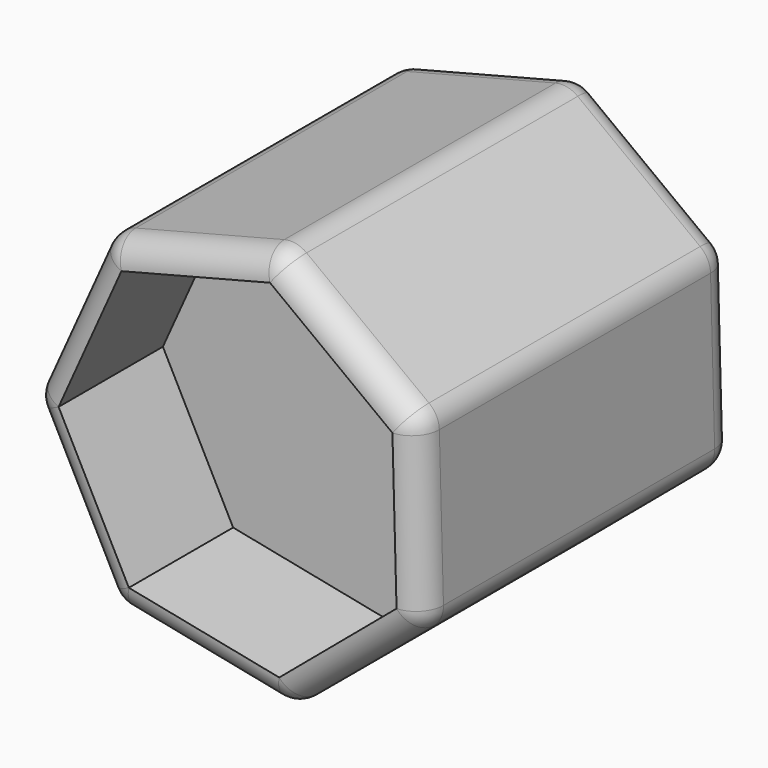
from build123d import *

# Parameters (mm, degrees)
F1_DEPTH     = 76.2
F2_F1_R      = 5.08
F2_F2_R      = 5.08
F2_F3_R      = 5.08
F2_F4_R      = 5.08
F3_T1_DEPTH  = 66.04
F3_T3_DEPTH  = 29.883199232
F3_T5_DEPTH  = 29.883199232
F3_T7_DEPTH  = 29.883199232
F3_T9_DEPTH  = 29.883199232
F3_T14_DEPTH = 5.08
F3_T20_DEPTH = 5.08
F3_T26_DEPTH = 5.08
F3_T32_DEPTH = 5.08
F3_T38_DEPTH = 5.08
F3_T44_DEPTH = 5.08
F3_T50_DEPTH = 5.08
F3_T56_DEPTH = 5.08
F3_T62_DEPTH = 5.08
F3_T68_DEPTH = 5.08
F5_DEPTH     = 25.4
F6_DEPTH     = 25.4


# Not quite as in the source:
# - a fillet or chamfer that OpenCascade refuses, or shapes differently, is made with other operations: its cross-section is extruded or revolved along the edge and cut away or added
# - a feature of the source that left no trace in its solid (it failed there, or was rolled back) is left out


with BuildPart() as f1:
    # F0 (on Front) → F1 (new body)
    with BuildSketch(Plane.XZ):
        Polygon((36.5605491077, -17.381725656), (35.6265013603, 17.381725656), (7.8649714404, 38.3261150914), (-25.8190423903, 29.6798902177), (-40.0607906887, -2.0461652844), (-24.1359465072, -32.9616845282), (9.9637576777, -39.7866509615), align=None)
    extrude(amount=F1_DEPTH)

    # F2: fillet of radius 5.08 on 4 edges, made by hand

    # F2_f1
    f2_f1_edges = [f1.edges().sort_by_distance(p)[0] for p in [
        (7.8649714404, -38.1, 38.3261150914),
    ]]
    fillet(f2_f1_edges, radius=F2_F1_R)

    # F2_f2
    f2_f2_edges = [f1.edges().sort_by_distance(p)[0] for p in [
        (-25.8190423903, -38.1, 29.6798902177),
    ]]
    fillet(f2_f2_edges, radius=F2_F2_R)

    # F2_f3
    f2_f3_edges = [f1.edges().sort_by_distance(p)[0] for p in [
        (-8.9770354749, 0, 34.0030026545),
    ]]
    fillet(f2_f3_edges, radius=F2_F3_R)

    # F2_f4
    f2_f4_edges = [f1.edges().sort_by_distance(p)[0] for p in [
        (-8.9770354749, -76.2, 34.0030026545),
    ]]
    fillet(f2_f4_edges, radius=F2_F4_R)

    # F3: fillet of radius 5.08 on 19 edges, made by hand

    # F3_s2 → F3_t1 (cut)
    with BuildSketch(Plane.XZ.offset(5.08)):
        with BuildLine():
            ThreePointArc((35.6922091389, 14.9362091735), (35.1301118192, 17.1260312252), (33.6735514536, 18.8551078331))
            Line((33.6735514536, 18.8551078331), (35.6265013603, 17.381725656))
            Line((35.6265013603, 17.381725656), (35.6922091389, 14.9362091735))
        make_face()
        with BuildLine():
            ThreePointArc((34.6895354607, -18.957852653), (36.0511453352, -17.1530555552), (36.4948413291, -14.9362091735))
            Line((36.4948413291, -14.9362091735), (36.5605491077, -17.381725656))
            Line((36.5605491077, -17.381725656), (34.6895354607, -18.957852653))
        make_face()
        with BuildLine():
            ThreePointArc((7.564934043, -39.3065326972), (9.8249311044, -39.245809579), (11.8347713247, -38.2105239645))
            Line((11.8347713247, -38.2105239645), (9.9637576777, -39.7866509615))
            Line((9.9637576777, -39.7866509615), (7.564934043, -39.3065326972))
        make_face()
        with BuildLine():
            ThreePointArc((-25.2562170056, -30.7868598483), (-23.79965664, -32.5159364562), (-21.7371228725, -33.4418027925))
            Line((-21.7371228725, -33.4418027925), (-24.1359465072, -32.9616845282))
            Line((-24.1359465072, -32.9616845282), (-25.2562170056, -30.7868598483))
        make_face()
        with BuildLine():
            ThreePointArc((-38.9405201903, -4.2209899644), (-39.50261751, -2.0311679128), (-39.0589215161, 0.1856784689))
            Line((-39.0589215161, 0.1856784689), (-40.0607906887, -2.0461652844))
            Line((-40.0607906887, -2.0461652844), (-38.9405201903, -4.2209899644))
        make_face()
    extrude(amount=F3_T1_DEPTH, mode=Mode.SUBTRACT)

    # F3_s4 → F3_t3 (cut)
    with BuildSketch(Plane(origin=(0.4273541338, 0, -15.9052946325), x_dir=(0, 1, 0), z_dir=(-0.026858978, 0, 0.9996392326))):
        with BuildLine():
            ThreePointArc((-76.2, -31.0005038658), (-74.7121024484, -34.5926063143), (-71.12, -36.0805038658))
            Line((-71.12, -36.0805038658), (-76.2, -36.0805038658))
            Line((-76.2, -36.0805038658), (-76.2, -31.0005038658))
        make_face()
        with BuildLine():
            ThreePointArc((0, -31.0005038658), (-1.4878975516, -34.5926063143), (-5.08, -36.0805038658))
            Line((-5.08, -36.0805038658), (0, -36.0805038658))
            Line((0, -36.0805038658), (0, -31.0005038658))
        make_face()
    extrude(amount=F3_T3_DEPTH, mode=Mode.SUBTRACT)

    # F3_s6 → F3_t5 (cut)
    with BuildSketch(Plane(origin=(-11.9052292748, 0, -10.0288703376), x_dir=(0, 1, 0), z_dir=(0.7648031243, 0, 0.6442640616))):
        with BuildLine():
            ThreePointArc((0, -31.7682459503), (-1.4878975516, -35.3603483987), (-5.08, -36.8482459503))
            Line((-5.08, -36.8482459503), (0, -36.8482459503))
            Line((0, -36.8482459503), (0, -31.7682459503))
        make_face()
        with BuildLine():
            ThreePointArc((-76.2, -31.7682459503), (-74.7121024484, -35.3603483987), (-71.12, -36.8482459503))
            Line((-71.12, -36.8482459503), (-76.2, -36.8482459503))
            Line((-76.2, -36.8482459503), (-76.2, -31.7682459503))
        make_face()
    extrude(amount=F3_T5_DEPTH, mode=Mode.SUBTRACT)

    # F3_s8 → F3_t7 (cut)
    with BuildSketch(Plane(origin=(-14.4644044829, 0, 2.8950126528), x_dir=(0, 1, 0), z_dir=(0.9805528748, 0, -0.1962550883))):
        with BuildLine():
            ThreePointArc((0, -31.9774768364), (-1.4878975516, -35.5695792849), (-5.08, -37.0574768364))
            Line((-5.08, -37.0574768364), (0, -37.0574768364))
            Line((0, -37.0574768364), (0, -31.9774768364))
        make_face()
        with BuildLine():
            ThreePointArc((-76.2, -31.9774768364), (-74.7121024484, -35.5695792849), (-71.12, -37.0574768364))
            Line((-71.12, -37.0574768364), (-76.2, -37.0574768364))
            Line((-76.2, -37.0574768364), (-76.2, -31.9774768364))
        make_face()
    extrude(amount=F3_T7_DEPTH, mode=Mode.SUBTRACT)

    # F3_s10 → F3_t9 (cut)
    with BuildSketch(Plane(origin=(-6.4473598679, 0, 12.5165104158), x_dir=(0, 1, 0), z_dir=(0.457926311, 0, -0.8889901539))):
        with BuildLine():
            ThreePointArc((-71.12, -36.5506413995), (-74.7121024484, -35.0627438479), (-76.2, -31.4706413995))
            Line((-76.2, -31.4706413995), (-76.2, -36.5506413995))
            Line((-76.2, -36.5506413995), (-71.12, -36.5506413995))
        make_face()
        with BuildLine():
            ThreePointArc((-5.08, -36.5506413995), (-1.4878975516, -35.0627438479), (0, -31.4706413995))
            Line((0, -31.4706413995), (0, -36.5506413995))
            Line((0, -36.5506413995), (-5.08, -36.5506413995))
        make_face()
    extrude(amount=F3_T9_DEPTH, mode=Mode.SUBTRACT)


with BuildPart() as f3_tool12:
    # F3_s13 → F3_t14 (new body)
    with BuildSketch(Plane.XZ.offset(71.12)):
        Polygon((30.6140418374, 14.7997655654), (35.6922091389, 14.9362091735), (35.6265013603, 17.381725656), (33.6735514536, 18.8551078331), align=None)
    extrude(amount=F3_T14_DEPTH)

    # F3_s15 → F3_t16 (revolve, cut)
    with BuildSketch(Plane(origin=(30.6140418374, -71.12, 14.7997655654), x_dir=(-0.8889901539, 0, -0.457926311), z_dir=(-0.457926311, 0, 0.8889901539))):
        with BuildLine():
            ThreePointArc((0, -5.08), (5.08, 0), (0, 5.08))
            Line((0, 5.08), (0, -5.08))
        make_face()
    revolve(axis=Axis((30.6140418374, -71.12, 14.7997655654), (0, -1, 0)), mode=Mode.SUBTRACT)


with BuildPart() as f1_1:
    add(f1.part)

    # F3_t11: cut F3_tool12
    add(f3_tool12.part, mode=Mode.SUBTRACT)


with BuildPart() as f3_tool18:
    # F3_s19 → F3_t20 (new body)
    with BuildSketch(Plane.XZ.offset(5.08)):
        Polygon((30.6140418374, 14.7997655654), (35.6922091389, 14.9362091735), (35.6265013603, 17.381725656), (33.6735514536, 18.8551078331), align=None)
    extrude(amount=-F3_T20_DEPTH)

    # F3_s21 → F3_t22 (revolve, cut)
    with BuildSketch(Plane(origin=(30.6140418374, -5.08, 14.7997655654), x_dir=(-0.8889901539, 0, -0.457926311), z_dir=(0.457926311, 0, -0.8889901539))):
        with BuildLine():
            ThreePointArc((0, -5.08), (5.08, 0), (0, 5.08))
            Line((0, 5.08), (0, -5.08))
        make_face()
    revolve(axis=Axis((30.6140418374, -5.08, 14.7997655654), (0, 1, 0)), mode=Mode.SUBTRACT)


with BuildPart() as f1_2:
    add(f1_1.part)

    # F3_t17: cut F3_tool18
    add(f3_tool18.part, mode=Mode.SUBTRACT)


with BuildPart() as f3_tool24:
    # F3_s25 → F3_t26 (new body)
    with BuildSketch(Plane.XZ.offset(5.08)):
        Polygon((-34.4244502085, -1.8947243046), (-38.9405201903, -4.2209899644), (-40.0607906887, -2.0461652844), (-39.0589215161, 0.1856784689), align=None)
    extrude(amount=-F3_T26_DEPTH)

    # F3_s27 → F3_t28 (revolve, cut)
    with BuildSketch(Plane(origin=(-34.4244502085, -5.08, -1.8947243046), x_dir=(0.9996392326, 0, 0.026858978), z_dir=(-0.026858978, 0, 0.9996392326))):
        with BuildLine():
            ThreePointArc((0, -5.08), (5.08, 0), (0, 5.08))
            Line((0, 5.08), (0, -5.08))
        make_face()
    revolve(axis=Axis((-34.4244502085, -5.08, -1.8947243046), (0, 1, 0)), mode=Mode.SUBTRACT)


with BuildPart() as f1_3:
    add(f1_2.part)

    # F3_t23: cut F3_tool24
    add(f3_tool24.part, mode=Mode.SUBTRACT)


with BuildPart() as f3_tool30:
    # F3_s31 → F3_t32 (new body)
    with BuildSketch(Plane.XZ.offset(71.12)):
        Polygon((-34.4244502085, -1.8947243046), (-38.9405201903, -4.2209899644), (-40.0607906887, -2.0461652844), (-39.0589215161, 0.1856784689), align=None)
    extrude(amount=F3_T32_DEPTH)

    # F3_s33 → F3_t34 (revolve, cut)
    with BuildSketch(Plane(origin=(-34.4244502085, -71.12, -1.8947243046), x_dir=(0.9996392326, 0, 0.026858978), z_dir=(0.026858978, 0, -0.9996392326))):
        with BuildLine():
            ThreePointArc((0, -5.08), (5.08, 0), (0, 5.08))
            Line((0, 5.08), (0, -5.08))
        make_face()
    revolve(axis=Axis((-34.4244502085, -71.12, -1.8947243046), (0, -1, 0)), mode=Mode.SUBTRACT)


with BuildPart() as f1_4:
    add(f1_3.part)

    # F3_t29: cut F3_tool30
    add(f3_tool30.part, mode=Mode.SUBTRACT)


with BuildPart() as f3_tool36:
    # F3_s37 → F3_t38 (new body)
    with BuildSketch(Plane.XZ.offset(71.12)):
        Polygon((31.4166740277, -15.0726527817), (36.4948413291, -14.9362091735), (36.5605491077, -17.381725656), (34.6895354607, -18.957852653), align=None)
    extrude(amount=F3_T38_DEPTH)

    # F3_s39 → F3_t40 (revolve, cut)
    with BuildSketch(Plane(origin=(31.4166740277, -71.12, -15.0726527817), x_dir=(-0.9122975015, 0, 0.409528105), z_dir=(0.409528105, 0, 0.9122975015))):
        with BuildLine():
            ThreePointArc((0, -5.08), (5.08, 0), (0, 5.08))
            Line((0, 5.08), (0, -5.08))
        make_face()
    revolve(axis=Axis((31.4166740277, -71.12, -15.0726527817), (0, -1, 0)), mode=Mode.SUBTRACT)


with BuildPart() as f1_5:
    add(f1_4.part)

    # F3_t35: cut F3_tool36
    add(f3_tool36.part, mode=Mode.SUBTRACT)


with BuildPart() as f3_tool42:
    # F3_s43 → F3_t44 (new body)
    with BuildSketch(Plane.XZ.offset(5.08)):
        Polygon((31.4166740277, -15.0726527817), (36.4948413291, -14.9362091735), (36.5605491077, -17.381725656), (34.6895354607, -18.957852653), align=None)
    extrude(amount=-F3_T44_DEPTH)

    # F3_s45 → F3_t46 (revolve, cut)
    with BuildSketch(Plane(origin=(31.4166740277, -5.08, -15.0726527817), x_dir=(-0.9122975015, 0, 0.409528105), z_dir=(-0.409528105, 0, -0.9122975015))):
        with BuildLine():
            ThreePointArc((0, -5.08), (5.08, 0), (0, 5.08))
            Line((0, 5.08), (0, -5.08))
        make_face()
    revolve(axis=Axis((31.4166740277, -5.08, -15.0726527817), (0, 1, 0)), mode=Mode.SUBTRACT)


with BuildPart() as f1_6:
    add(f1_5.part)

    # F3_t41: cut F3_tool42
    add(f3_tool42.part, mode=Mode.SUBTRACT)


with BuildPart() as f3_tool48:
    # F3_s49 → F3_t50 (new body)
    with BuildSketch(Plane.XZ.offset(5.08)):
        Polygon((8.5619098917, -34.3253240931), (7.564934043, -39.3065326972), (9.9637576777, -39.7866509615), (11.8347713247, -38.2105239645), align=None)
    extrude(amount=-F3_T50_DEPTH)

    # F3_s51 → F3_t52 (revolve, cut)
    with BuildSketch(Plane(origin=(8.5619098917, -5.08, -34.3253240931), x_dir=(-0.248626223, 0, 0.9685995051), z_dir=(-0.9685995051, 0, -0.248626223))):
        with BuildLine():
            ThreePointArc((0, -5.08), (5.08, 0), (0, 5.08))
            Line((0, 5.08), (0, -5.08))
        make_face()
    revolve(axis=Axis((8.5619098917, -5.08, -34.3253240931), (0, 1, 0)), mode=Mode.SUBTRACT)


with BuildPart() as f1_7:
    add(f1_6.part)

    # F3_t47: cut F3_tool48
    add(f3_tool48.part, mode=Mode.SUBTRACT)


with BuildPart() as f3_tool54:
    # F3_s55 → F3_t56 (new body)
    with BuildSketch(Plane.XZ.offset(71.12)):
        Polygon((8.5619098917, -34.3253240931), (7.564934043, -39.3065326972), (9.9637576777, -39.7866509615), (11.8347713247, -38.2105239645), align=None)
    extrude(amount=F3_T56_DEPTH)

    # F3_s57 → F3_t58 (revolve, cut)
    with BuildSketch(Plane(origin=(8.5619098917, -71.12, -34.3253240931), x_dir=(-0.248626223, 0, 0.9685995051), z_dir=(0.9685995051, 0, 0.248626223))):
        with BuildLine():
            ThreePointArc((0, -5.08), (5.08, 0), (0, 5.08))
            Line((0, 5.08), (0, -5.08))
        make_face()
    revolve(axis=Axis((8.5619098917, -71.12, -34.3253240931), (0, -1, 0)), mode=Mode.SUBTRACT)


with BuildPart() as f1_8:
    add(f1_7.part)

    # F3_t53: cut F3_tool54
    add(f3_tool54.part, mode=Mode.SUBTRACT)


with BuildPart() as f3_tool60:
    # F3_s61 → F3_t62 (new body)
    with BuildSketch(Plane.XZ.offset(5.08)):
        Polygon((-20.7401470239, -28.4605941885), (-21.7371228725, -33.4418027925), (-24.1359465072, -32.9616845282), (-25.2562170056, -30.7868598483), align=None)
    extrude(amount=-F3_T62_DEPTH)

    # F3_s63 → F3_t64 (revolve, cut)
    with BuildSketch(Plane(origin=(-20.7401470239, -5.08, -28.4605941885), x_dir=(0.6022656725, 0, 0.798295722), z_dir=(-0.798295722, 0, 0.6022656725))):
        with BuildLine():
            ThreePointArc((0, -5.08), (5.08, 0), (0, 5.08))
            Line((0, 5.08), (0, -5.08))
        make_face()
    revolve(axis=Axis((-20.7401470239, -5.08, -28.4605941885), (0, 1, 0)), mode=Mode.SUBTRACT)


with BuildPart() as f1_9:
    add(f1_8.part)

    # F3_t59: cut F3_tool60
    add(f3_tool60.part, mode=Mode.SUBTRACT)


with BuildPart() as f3_tool66:
    # F3_s67 → F3_t68 (new body)
    with BuildSketch(Plane.XZ.offset(71.12)):
        Polygon((-20.7401470239, -28.4605941885), (-21.7371228725, -33.4418027925), (-24.1359465072, -32.9616845282), (-25.2562170056, -30.7868598483), align=None)
    extrude(amount=F3_T68_DEPTH)

    # F3_s69 → F3_t70 (revolve, cut)
    with BuildSketch(Plane(origin=(-20.7401470239, -71.12, -28.4605941885), x_dir=(0.6022656725, 0, 0.798295722), z_dir=(0.798295722, 0, -0.6022656725))):
        with BuildLine():
            ThreePointArc((0, -5.08), (5.08, 0), (0, 5.08))
            Line((0, 5.08), (0, -5.08))
        make_face()
    revolve(axis=Axis((-20.7401470239, -71.12, -28.4605941885), (0, -1, 0)), mode=Mode.SUBTRACT)


with BuildPart() as f1_10:
    add(f1_9.part)

    # F3_t65: cut F3_tool66
    add(f3_tool66.part, mode=Mode.SUBTRACT)

    # F5 (cut): a face of the model
    f5_faces = [f1_10.faces().sort_by_distance(p)[0] for p in [
        (0, -76.2, -0.9697850665),
    ]]
    extrude(f5_faces, amount=-F5_DEPTH, mode=Mode.SUBTRACT)

    # F6 (cut): a face of the model
    f6_faces = [f1_10.faces().sort_by_distance(p)[0] for p in [
        (0, 0, -0.9697850665),
    ]]
    extrude(f6_faces, amount=-F6_DEPTH, mode=Mode.SUBTRACT)


solid = f1_10.part
